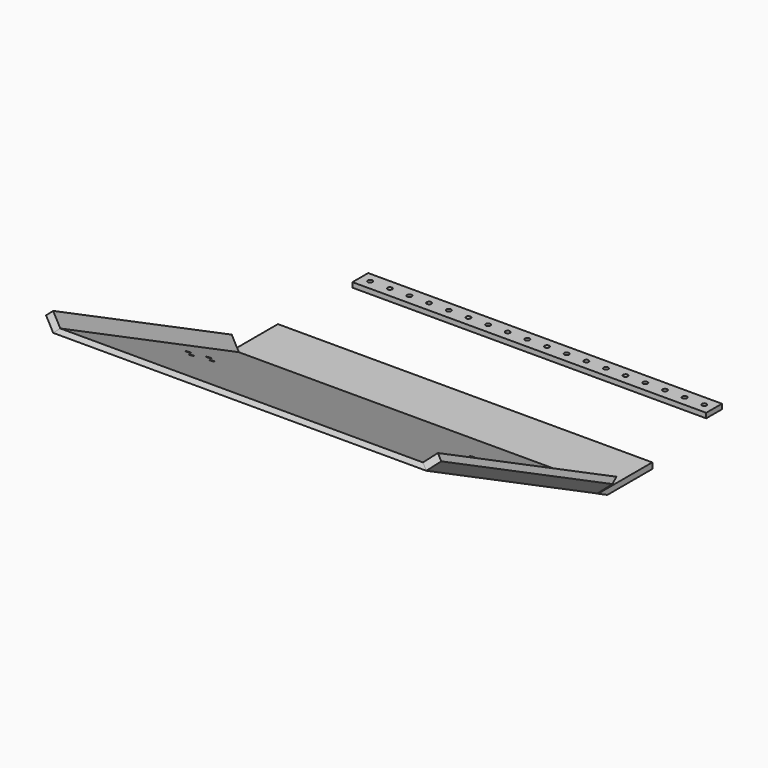
from build123d import *

# Parameters (mm, degrees)
F0_W        = 45.72
F0_H        = 4.7625
F1_DEPTH    = 304.8
F2_T4_DEPTH = 227.6952804604
F2_T9_DEPTH = 227.6952804604
F3_DEPTH    = 12.7
F4_DEPTH    = 12.7
F5_W        = 288
F5_H        = 16
F6_DEPTH    = 4
F7_R        = 1.905
F8_DEPTH    = 4
F9_R        = 1.905
F10_DEPTH   = 4.2595255188


# Not quite as in the source:
# - a fillet or chamfer that OpenCascade refuses, or shapes differently, is made with other operations: its cross-section is extruded or revolved along the edge and cut away or added


with BuildPart() as f1:
    # F0 (on Right) → F1 (new body)
    with BuildSketch(Plane.YZ):
        with Locations((-22.86, 2.38125)):
            Rectangle(F0_W, F0_H)
        Polygon((-229.3650022503, 91.8423295021), (-45.72, 0), (-45.72, 4.7625), (-227.4597554672, 95.6520003987), align=None)
    extrude(amount=F1_DEPTH)

    # F2: chamfer of 4.7625 on 2 edges, made by hand


with BuildPart() as f2_tool2:
    # F2_s3 → F2_t4 (new body)
    with BuildSketch(Plane(origin=(0, -27.523938077, 13.764940832), x_dir=(1, 0, 0), z_dir=(0, -0.8943885604, 0.4472908484))):
        Polygon((300.0375, -16.1906120709), (304.8, -20.9531120709), (304.8, -16.1906120709), align=None)
    extrude(amount=F2_T4_DEPTH)

    split(bisect_by=Plane.XY.offset(4.7625), keep=Keep.TOP)


with BuildPart() as f1_1:
    add(f1.part)

    # F2_t1: cut F2_tool2
    add(f2_tool2.part, mode=Mode.SUBTRACT)


with BuildPart() as f2_tool7:
    # F2_s8 → F2_t9 (new body)
    with BuildSketch(Plane(origin=(0, -27.523938077, 13.764940832), x_dir=(1, 0, 0), z_dir=(0, -0.8943885604, 0.4472908484))):
        Polygon((4.7625, -16.1906120709), (0, -20.9531120709), (0, -16.1906120709), align=None)
    extrude(amount=F2_T9_DEPTH)

    split(bisect_by=Plane.XY.offset(4.7625), keep=Keep.TOP)


with BuildPart() as f1_2:
    add(f1_1.part)

    # F2_t6: cut F2_tool7
    add(f2_tool7.part, mode=Mode.SUBTRACT)

    # F3 (add): a face of the model
    f3_faces = [f1_2.faces().sort_by_distance(p)[0] for p in [
        (302.1520659552, -139.4265390225, 49.2616283991),
    ]]
    extrude(f3_faces, amount=F3_DEPTH)

    # F4 (add): a face of the model
    f4_faces = [f1_2.faces().sort_by_distance(p)[0] for p in [
        (2.6479340448, -139.4265390225, 49.2616283991),
    ]]
    extrude(f4_faces, amount=F4_DEPTH)

    # F9 (on face) → F10 (cut, through all)
    with BuildSketch(Plane(origin=(0, -9.1471593928, -18.2903691182), x_dir=(1, 0, 0), z_dir=(0, -0.4472908484, -0.8943885604))):
        with Locations((36.7665, 122.1426676457)):
            Circle(F9_R)
        with Locations((46.5455, 131.9216676457)):
            Circle(F9_R)
        with Locations((36.7665, 141.7006676457)):
            Circle(F9_R)
        with Locations((26.9875, 131.9216676457)):
            Circle(F9_R)
        with Locations((277.8125, 131.9216676457)):
            Circle(F9_R)
        with Locations((258.2545, 131.9216676457)):
            Circle(F9_R)
        with Locations((268.0335, 122.1426676457)):
            Circle(F9_R)
        with Locations((268.0335, 141.7006676457)):
            Circle(F9_R)
    extrude(amount=-F10_DEPTH, mode=Mode.SUBTRACT)


with BuildPart() as f6:
    # F5 (on Top) → F6 (new body)
    with BuildSketch(Plane.XY):
        with Locations((144, 83.8868339212)):
            Rectangle(F5_W, F5_H)
    extrude(amount=F6_DEPTH)

    # F7 (on face) → F8 (cut, through all)
    with BuildSketch(Plane.XY.offset(4)):
        with Locations((8, 83.8868339212)):
            Circle(F7_R)
        with Locations((24, 83.8868339212)):
            Circle(F7_R)
        with Locations((40, 83.8868339212)):
            Circle(F7_R)
        with Locations((56, 83.8868339212)):
            Circle(F7_R)
        with Locations((72, 83.8868339212)):
            Circle(F7_R)
        with Locations((88, 83.8868339212)):
            Circle(F7_R)
        with Locations((104, 83.8868339212)):
            Circle(F7_R)
        with Locations((120, 83.8868339212)):
            Circle(F7_R)
        with Locations((136, 83.8868339212)):
            Circle(F7_R)
        with Locations((152, 83.8868339212)):
            Circle(F7_R)
        with Locations((168, 83.8868339212)):
            Circle(F7_R)
        with Locations((184, 83.8868339212)):
            Circle(F7_R)
        with Locations((200, 83.8868339212)):
            Circle(F7_R)
        with Locations((216, 83.8868339212)):
            Circle(F7_R)
        with Locations((232, 83.8868339212)):
            Circle(F7_R)
        with Locations((248, 83.8868339212)):
            Circle(F7_R)
        with Locations((264, 83.8868339212)):
            Circle(F7_R)
        with Locations((280, 83.8868339212)):
            Circle(F7_R)
    extrude(amount=-F8_DEPTH, mode=Mode.SUBTRACT)


solid = Compound([f1_2.part, f6.part])
